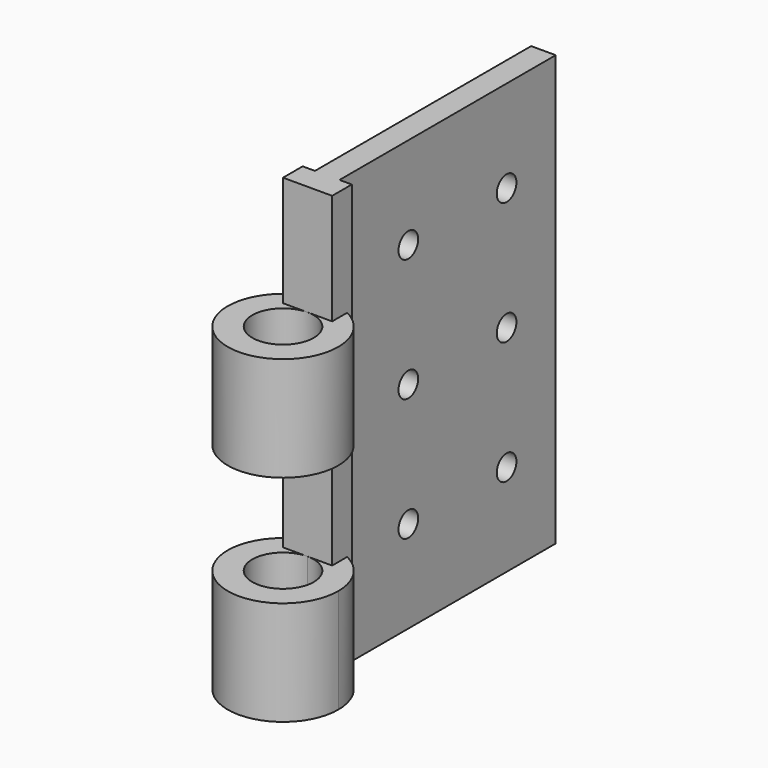
from build123d import *

# Parameters (mm, degrees)
F0_W     = 2
F0_H     = 35
F1_DEPTH = 22
F2_R     = 1
F3_DEPTH = 25
F4_W     = 1
F4_H     = 35
F4_W_2   = 2
F5_DEPTH = 2
F8_R     = 4.5
F8_R_2   = 2.5
F9_DEPTH = 8.5


# Not quite as in the source:
# - a feature names something its author has since deleted; it is built from what else it names


with BuildPart() as f1:
    # F0 (on Front) → F1 (new body)
    with BuildSketch(Plane.XZ):
        Rectangle(F0_W, F0_H)
    extrude(amount=F1_DEPTH)

    # F2 (on face) → F3 (cut)
    with BuildSketch(Plane(origin=(-1, 0, 0), x_dir=(0, -1, 0), z_dir=(-1, 0, 0))):
        with Locations((5, 10)):
            Circle(F2_R)
        with Locations((15, 10)):
            Circle(F2_R)
        with Locations((15, 0)):
            Circle(F2_R)
        with Locations((5, 0)):
            Circle(F2_R)
        with Locations((5, -10)):
            Circle(F2_R)
        with Locations((15, -10)):
            Circle(F2_R)
    extrude(amount=-F3_DEPTH, mode=Mode.SUBTRACT)

    # F4 (on face) → F5 (join)
    with BuildSketch(Plane.XZ.offset(22)):
        with Locations((-1.5, 0)):
            Rectangle(F4_W, F4_H)
        with Locations((1.5, 0)):
            Rectangle(F4_W, F4_H)
        Rectangle(F4_W_2, F4_H)
    extrude(amount=F5_DEPTH)

    # F8 (on offset) + F6 (on face) → F9 (join)
    with BuildSketch(Plane(origin=(0, 0, 0), x_dir=(1, 0, 0), z_dir=(0, 0, -1))):
        with Locations((0, 26.5)):
            Circle(F8_R)
        with Locations((0, 26.5)):
            Circle(F8_R_2, mode=Mode.SUBTRACT)
    with BuildSketch(Plane(origin=(0, 0, -17.5), x_dir=(1, 0, 0), z_dir=(0, 0, -1))):
        with BuildLine():
            Line((-2, 24), (0, 24))
            Line((0, 24), (2, 24))
            Line((2, 24), (2, 22.4688711259))
            ThreePointArc((2, 22.4688711259), (3.8242646352, 24.1282917549), (4.5, 26.5))
            ThreePointArc((4.5, 26.5), (-2.3717082451, 30.3242646352), (-2, 22.4688711259))
            Line((-2, 22.4688711259), (-2, 24))
        make_face()
        with BuildLine():
            ThreePointArc((0, 24), (-1.767766953, 28.267766953), (2.5, 26.5))
            ThreePointArc((2.5, 26.5), (1.767766953, 24.732233047), (0, 24))
        make_face(mode=Mode.SUBTRACT)
    extrude(amount=-F9_DEPTH)


solid = f1.part
